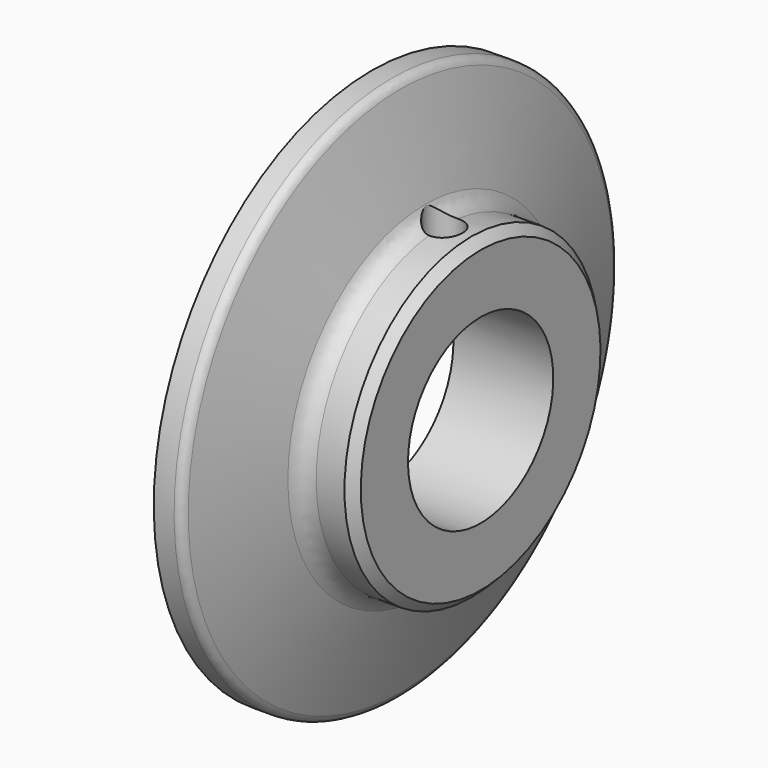
from build123d import *

# Parameters (mm, degrees)
F2_SIZE  = 1
F3_R     = 0.99999
F4_R     = 2
F5_R     = 2
F6_DEPTH = 30.0010001


# Not quite as in the source:
# - a fillet or chamfer is up to 0.001 mm smaller than in the source, because OpenCascade refuses the exact size


with BuildPart() as f1:
    # F0 (on Front) → F1 (revolve)
    with BuildSketch(Plane.XZ):
        Polygon((0, 30), (0, 20), (1, 20), (1, 10), (12, 10), (12, 17.5), (6.3493649054, 17.5), (3, 30), align=None)
    revolve(axis=Axis((7.1844396027, 0, 0), (1, 0, 0)))

    # F2
    f2_edges = [f1.edges().sort_by_distance(p)[0] for p in [
        (12, 0, -17.5),
    ]]
    chamfer(f2_edges, length=F2_SIZE)

    # F3 (radius 1 in the source; OpenCascade refuses exactly that, so slightly less here)
    f3_edges = [f1.edges().sort_by_distance(p)[0] for p in [
        (3, 0, -30),
        (1, 0, -20),
    ]]
    fillet(f3_edges, radius=F3_R)

    # F4
    f4_edges = [f1.edges().sort_by_distance(p)[0] for p in [
        (6.349365, 0, -17.5),
    ]]
    fillet(f4_edges, radius=F4_R)

    # F5 (on Top) → F6 (cut, through all)
    with BuildSketch(Plane.XY):
        with Locations((8, 0)):
            Circle(F5_R)
    extrude(amount=F6_DEPTH, mode=Mode.SUBTRACT)


solid = f1.part
